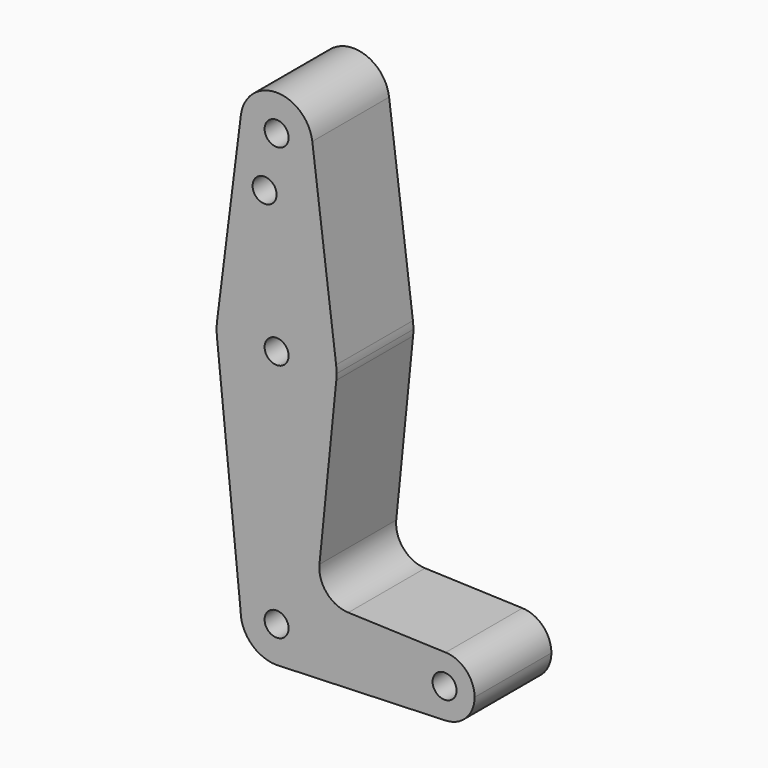
from build123d import *

# Parameters (mm, degrees)
F2_R     = 3.175
F3_DEPTH = 25.4


# Not quite as in the source:
# - a feature names something its author has since deleted; it is built from what else it names


with BuildPart() as f3:
    # F2 (on Front) → F3 (new body)
    with BuildSketch(Plane.XZ):
        with BuildLine():
            ThreePointArc((15.7504884308, 65.4843737526), (6.286e-07, 79.375), (-15.7504882737, 65.484375))
            ThreePointArc((-15.7504882737, 65.484375), (-15.8738192656, 63.6936154008), (-15.7942028036, 61.9003804205))
            ThreePointArc((-15.7942028036, 61.9003804205), (0.0060905531, 47.6250011683), (15.7954255641, 61.9125))
            ThreePointArc((15.7954255641, 61.9125), (15.8550939106, 62.7052534459), (15.875, 63.5))
            ThreePointArc((15.875, 63.5), (15.8438415297, 64.4941381092), (15.7504884308, 65.4843737526))
        make_face()
        with Locations((0, 63.5)):
            Circle(F2_R, mode=Mode.SUBTRACT)
        with BuildLine():
            Line((-9.4502929642, 115.490625), (-15.7504882737, 65.484375))
            ThreePointArc((-15.7504882737, 65.484375), (6.286e-07, 79.375), (15.7504884308, 65.4843737526))
            Line((15.7504884308, 65.4843737526), (9.4502929642, 115.490625))
            ThreePointArc((9.4502929642, 115.490625), (9.5063048942, 114.896483242), (9.525, 114.3))
            ThreePointArc((9.525, 114.3), (-0.596483242, 104.7936951058), (-9.4502929642, 115.490625))
        make_face()
        with Locations((-3.175, 100.0252)):
            Circle(F2_R, mode=Mode.SUBTRACT)
        with BuildLine():
            ThreePointArc((15.7954255641, 61.9125), (0.0060905531, 47.6250011683), (-15.7942028036, 61.9003804205))
            Line((-15.7942028036, 61.9003804205), (-9.525, 0))
            ThreePointArc((-9.525, 0), (0, 9.525), (9.525, 0))
            ThreePointArc((9.525, 0), (6.9705567315, -6.4912990883), (0.6773435479, -9.500885786))
            Line((0.6773435479, -9.500885786), (44.7324052746, -7.9324746146))
            ThreePointArc((44.7324052746, -7.9324746146), (36.5125, 0), (44.7324052746, 7.9324746146))
            Line((44.7324052746, 7.9324746146), (18.968327868, 8.8497055806))
            ThreePointArc((18.968327868, 8.8497055806), (13.2612039825, 11.5674628959), (11.3408358685, 17.5898921545))
            Line((11.3408358685, 17.5898921545), (15.7954255641, 61.9125))
        make_face()
        with BuildLine():
            ThreePointArc((9.4502929642, 115.490625), (0, 123.825), (-9.4502929642, 115.490625))
            ThreePointArc((-9.4502929642, 115.490625), (-0.596483242, 104.7936951058), (9.525, 114.3))
            ThreePointArc((9.525, 114.3), (9.5063048942, 114.896483242), (9.4502929642, 115.490625))
        make_face()
        with Locations((0, 114.3)):
            Circle(F2_R, mode=Mode.SUBTRACT)
        with BuildLine():
            ThreePointArc((9.525, 0), (0, 9.525), (-9.525, 0))
            ThreePointArc((-9.525, 0), (-6.7351920908, -6.7351920908), (0, -9.525))
            Line((0, -9.525), (0.6773435479, -9.500885786))
            ThreePointArc((0.6773435479, -9.500885786), (6.9705567315, -6.4912990883), (9.525, 0))
        make_face()
        Circle(F2_R, mode=Mode.SUBTRACT)
        with BuildLine():
            Line((0.6773435479, -9.500885786), (0, -9.525))
            ThreePointArc((0, -9.525), (0.3388863295, -9.5189695375), (0.6773435479, -9.500885786))
        make_face()
        with BuildLine():
            ThreePointArc((52.3875, 0), (50.1616327839, 5.5119104847), (44.7324052746, 7.9324746146))
            ThreePointArc((44.7324052746, 7.9324746146), (36.5125, 0), (44.7324052746, -7.9324746146))
            ThreePointArc((44.7324052746, -7.9324746146), (50.1616327839, -5.5119104847), (52.3875, 0))
        make_face()
        with Locations((44.45, 0)):
            Circle(F2_R, mode=Mode.SUBTRACT)
    extrude(amount=F3_DEPTH)


solid = f3.part
